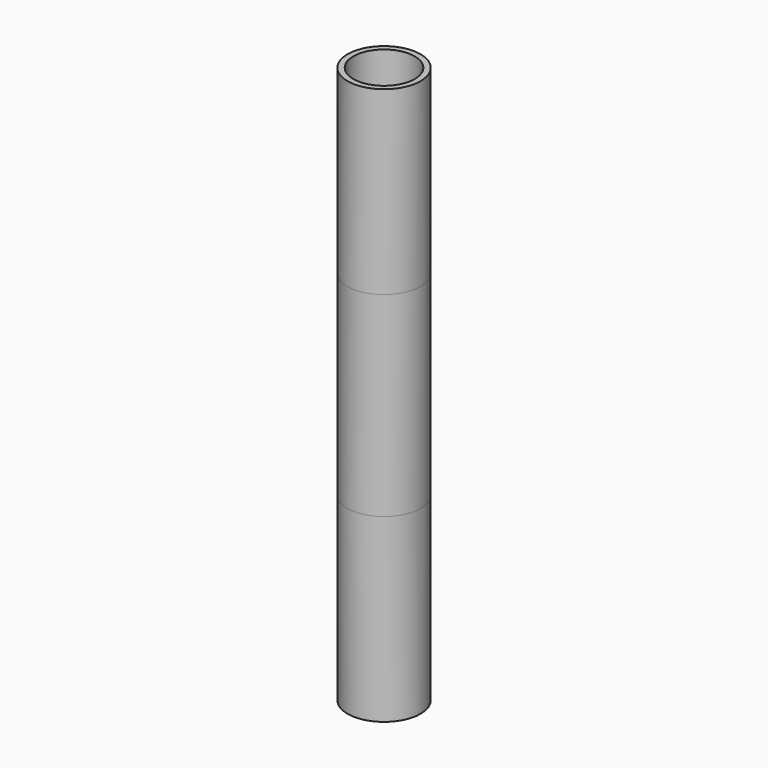
from build123d import *

# Parameters (mm, degrees)
F0_R          = 30.1625
F0_R_2        = 25.4
F1_DEPTH      = 304.8
F1_DEPTH_BACK = 6.125


# Not quite as in the source:
# - a pattern or mirror of a feature is missing from the dataset's text; its kind, count and spacing are read off the source's solid


with BuildPart() as f1:
    # F0 (on Top) → F1 (new body, two sides)
    with BuildSketch(Plane.XY) as f1_sk:
        Circle(F0_R)
        Circle(F0_R_2, mode=Mode.SUBTRACT)
    extrude(amount=F1_DEPTH)
    extrude(f1_sk.sketch, amount=-F1_DEPTH_BACK)

    # F1_copies: F1 across plane


with BuildPart() as f1_1:
    add(f1.part)
    add(f1.part.mirror(Plane(origin=(0, 0, 74.6125), x_dir=(-1, 0, 0), z_dir=(0, 0, -1))))


solid = f1_1.part
